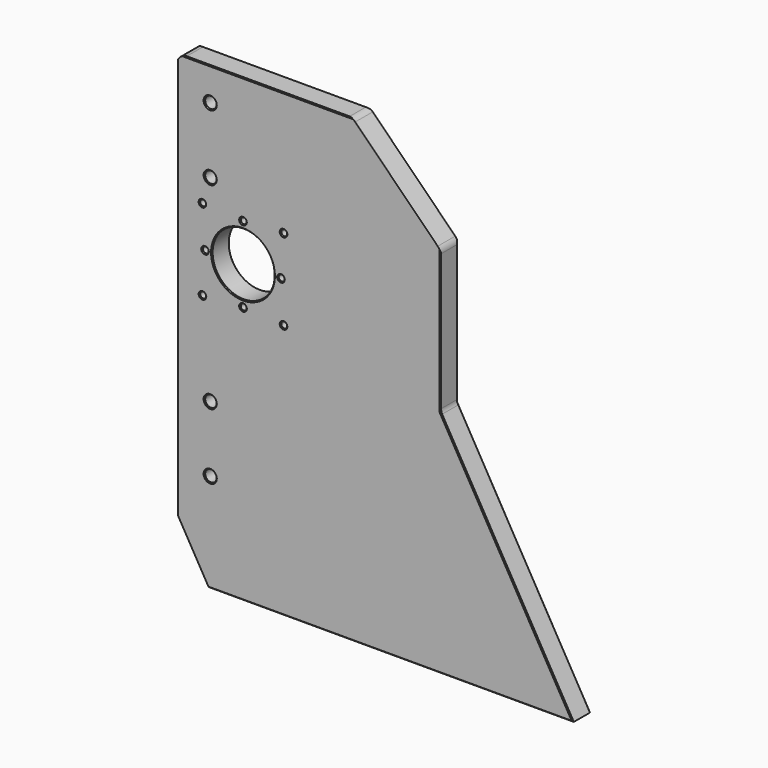
from build123d import *

# Parameters (mm, degrees)
F0_R         = 3.302
F0_R_2       = 1.7
F0_R_3       = 18
F1_DEPTH     = 12.7
F2_SIZE      = 0.508
F3_T1_DEPTH  = 272.9669915773
F4_T4_DEPTH  = 18.4899094878
F4_T10_DEPTH = 18.4899094878
F4_T16_DEPTH = 18.4899094878
F4_T24_DEPTH = 18.4899094878
F4_T30_DEPTH = 18.4899094878
F4_T33_DEPTH = 22.2050244844
F4_T35_DEPTH = 18.4899094878
F4_T37_DEPTH = 37.084


# Not quite as in the source:
# - a fillet or chamfer that OpenCascade refuses, or shapes differently, is made with other operations: its cross-section is extruded or revolved along the edge and cut away or added


with BuildPart() as f1:
    # F0 (on Front) → F1 (new body)
    with BuildSketch(Plane.XZ):
        Polygon((44.9265169831, 0), (44.9265169831, 133.35), (-107.4734830169, 133.35), (-107.4734830169, -102.6728227735), (-89.7620064872, -133.35), (121.9161753795, -133.35), align=None)
        with Locations((-88.4234830169, -76.1876442577)):
            Circle(F0_R, mode=Mode.SUBTRACT)
        with Locations((-88.4234830169, -38.0876442577)):
            Circle(F0_R, mode=Mode.SUBTRACT)
        with Locations((-92.9194827628, 14.6180932346)):
            Circle(F0_R_2, mode=Mode.SUBTRACT)
        with Locations((-69.4244827628, 16.1130932346)):
            Circle(F0_R_2, mode=Mode.SUBTRACT)
        with Locations((-45.9294827628, 14.6180932346)):
            Circle(F0_R_2, mode=Mode.SUBTRACT)
        with Locations((-91.4244827628, 38.1130932346)):
            Circle(F0_R_2, mode=Mode.SUBTRACT)
        with Locations((-69.4244827628, 38.1130932346)):
            Circle(F0_R_3, mode=Mode.SUBTRACT)
        with Locations((-92.9194827628, 61.6080932346)):
            Circle(F0_R_2, mode=Mode.SUBTRACT)
        with Locations((-69.4244827628, 60.1130932346)):
            Circle(F0_R_2, mode=Mode.SUBTRACT)
        with Locations((-47.4244827628, 38.1130932346)):
            Circle(F0_R_2, mode=Mode.SUBTRACT)
        with Locations((-45.9294827628, 61.6080932346)):
            Circle(F0_R_2, mode=Mode.SUBTRACT)
        with Locations((-88.4234830169, 76.2)):
            Circle(F0_R, mode=Mode.SUBTRACT)
        with Locations((-88.4234830169, 114.3)):
            Circle(F0_R, mode=Mode.SUBTRACT)
    extrude(amount=F1_DEPTH)

    # F2
    f2_edges = [f1.edges().sort_by_distance(p)[0] for p in [
        (44.926517, -12.7, 66.675),
        (-31.273483, -12.7, 133.35),
        (-107.473483, -12.7, 15.338589),
        (-98.617745, -12.7, -118.011411),
        (16.077084, -12.7, -133.35),
        (83.421346, -12.7, -66.675),
        (-91.725483, -12.7, -76.187644),
        (-91.725483, -12.7, -38.087644),
        (-94.619483, -12.7, 14.618093),
        (-71.124483, -12.7, 16.113093),
        (-47.629483, -12.7, 14.618093),
        (-93.124483, -12.7, 38.113093),
        (-87.424483, -12.7, 38.113093),
        (-94.619483, -12.7, 61.608093),
        (-71.124483, -12.7, 60.113093),
        (-49.124483, -12.7, 38.113093),
        (-47.629483, -12.7, 61.608093),
        (-91.725483, -12.7, 76.2),
        (-91.725483, -12.7, 114.3),
        (44.926517, 0, 66.675),
        (-31.273483, 0, 133.35),
        (-107.473483, 0, 15.338589),
        (-98.617745, 0, -118.011411),
        (16.077084, 0, -133.35),
        (83.421346, 0, -66.675),
        (-91.725483, 0, -76.187644),
        (-91.725483, 0, -38.087644),
        (-94.619483, 0, 14.618093),
        (-71.124483, 0, 16.113093),
        (-47.629483, 0, 14.618093),
        (-93.124483, 0, 38.113093),
        (-87.424483, 0, 38.113093),
        (-94.619483, 0, 61.608093),
        (-71.124483, 0, 60.113093),
        (-49.124483, 0, 38.113093),
        (-47.629483, 0, 61.608093),
        (-91.725483, 0, 76.2),
        (-91.725483, 0, 114.3),
    ]]
    chamfer(f2_edges, length=F2_SIZE)

    # F3: chamfer of 50.8 on 1 edges, made by hand

    # F3_s2 → F3_t1 (cut)
    with BuildSketch(Plane.XZ.offset(-130.1334957887)):
        Polygon((44.9265169831, 82.55), (-5.8734830169, 133.35), (44.9265169831, 133.35), align=None)
    extrude(amount=F3_T1_DEPTH, mode=Mode.SUBTRACT)

    # F4: fillet of radius 5.08 on 5 edges, made by hand


with BuildPart() as f4_tool2:
    # F4_s3 → F4_t4 (new body)
    with BuildSketch(Plane.XZ.offset(-2.8949547439)):
        with BuildLine():
            ThreePointArc((44.9265169831, 1.3611818976), (45.0996137855, 0.0463811484), (45.6071079319, -1.1788181024))
            Line((45.6071079319, -1.1788181024), (44.9265169831, 0))
            Line((44.9265169831, 0), (44.9265169831, 1.3611818976))
        make_face()
    extrude(amount=F4_T4_DEPTH)

    split(bisect_by=Plane(origin=(22.2092584915, 22.2092584915, 0), x_dir=(0, 0, 1), z_dir=(0.7071067812, 0.7071067812, 0)), keep=Keep.TOP)

    split(bisect_by=Plane(origin=(16.6274734161, 19.1997525055, 9.5998762527), x_dir=(0.755928946, -0.6546536707, 0), z_dir=(-0.6123724357, -0.7071067812, -0.3535533906)), keep=Keep.TOP)


with BuildPart() as f1_1:
    add(f1.part)

    # F4_t1: union F4_tool2
    add(f4_tool2.part)


with BuildPart() as f4_tool8:
    # F4_s9 → F4_t10 (new body)
    with BuildSketch(Plane.XZ.offset(-2.8949547439)):
        with BuildLine():
            ThreePointArc((44.9265169831, 1.3611818976), (45.0996137855, 0.0463811484), (45.6071079319, -1.1788181024))
            Line((45.6071079319, -1.1788181024), (44.9265169831, 0))
            Line((44.9265169831, 0), (44.9265169831, 1.3611818976))
        make_face()
    extrude(amount=F4_T10_DEPTH)

    split(bisect_by=Plane(origin=(22.2092584915, 22.2092584915, 0), x_dir=(0, 0, 1), z_dir=(-0.7071067812, -0.7071067812, 0)), keep=Keep.TOP)

    split(bisect_by=Plane(origin=(16.6274734161, 19.1997525055, 9.5998762527), x_dir=(-0.755928946, 0.6546536707, 0), z_dir=(0.6123724357, 0.7071067812, 0.3535533906)), keep=Keep.TOP)


with BuildPart() as f1_2:
    add(f1_1.part)

    # F4_t7: union F4_tool8
    add(f4_tool8.part)


with BuildPart() as f4_tool14:
    # F4_s15 → F4_t16 (new body)
    with BuildSketch(Plane.XZ.offset(-2.8949547439)):
        with BuildLine():
            ThreePointArc((44.9265169831, 1.3611818976), (45.0996137855, 0.0463811484), (45.6071079319, -1.1788181024))
            Line((45.6071079319, -1.1788181024), (44.9265169831, 0))
            Line((44.9265169831, 0), (44.9265169831, 1.3611818976))
        make_face()
    extrude(amount=F4_T16_DEPTH)

    split(bisect_by=Plane(origin=(22.2092584915, 22.2092584915, 0), x_dir=(0, 0, 1), z_dir=(-0.7071067812, -0.7071067812, 0)), keep=Keep.TOP)

    split(bisect_by=Plane(origin=(28.5592584915, -28.5592584915, 0), x_dir=(0, 0, 1), z_dir=(-0.7071067812, 0.7071067812, 0)), keep=Keep.TOP)

    split(bisect_by=Plane(origin=(16.6274734161, 19.1997525055, 9.5998762527), x_dir=(0.755928946, -0.6546536707, 0), z_dir=(-0.6123724357, -0.7071067812, -0.3535533906)), keep=Keep.TOP)

    split(bisect_by=Plane(origin=(22.1267347301, -25.5497525055, 12.7748762527), x_dir=(-0.755928946, -0.6546536707, 0), z_dir=(-0.6123724357, 0.7071067812, -0.3535533906)), keep=Keep.TOP)


with BuildPart() as f1_3:
    add(f1_2.part)

    # F4_t13: union F4_tool14
    add(f4_tool14.part)


with BuildPart() as f4_tool22:
    # F4_s23 → F4_t24 (new body)
    with BuildSketch(Plane.XZ.offset(-2.8949547439)):
        with BuildLine():
            ThreePointArc((44.9265169831, 1.3611818976), (45.0996137855, 0.0463811484), (45.6071079319, -1.1788181024))
            Line((45.6071079319, -1.1788181024), (44.9265169831, 0))
            Line((44.9265169831, 0), (44.9265169831, 1.3611818976))
        make_face()
    extrude(amount=F4_T24_DEPTH)

    split(bisect_by=Plane(origin=(28.5592584915, -28.5592584915, 0), x_dir=(0, 0, 1), z_dir=(0.7071067812, -0.7071067812, 0)), keep=Keep.TOP)

    split(bisect_by=Plane(origin=(22.1267347301, -25.5497525055, 12.7748762527), x_dir=(-0.755928946, -0.6546536707, 0), z_dir=(-0.6123724357, 0.7071067812, -0.3535533906)), keep=Keep.TOP)


with BuildPart() as f1_4:
    add(f1_3.part)

    # F4_t21: union F4_tool22
    add(f4_tool22.part)


with BuildPart() as f4_tool28:
    # F4_s29 → F4_t30 (new body)
    with BuildSketch(Plane.XZ.offset(-2.8949547439)):
        with BuildLine():
            ThreePointArc((44.9265169831, 1.3611818976), (45.0996137855, 0.0463811484), (45.6071079319, -1.1788181024))
            Line((45.6071079319, -1.1788181024), (44.9265169831, 0))
            Line((44.9265169831, 0), (44.9265169831, 1.3611818976))
        make_face()
    extrude(amount=F4_T30_DEPTH)

    split(bisect_by=Plane(origin=(28.5592584915, -28.5592584915, 0), x_dir=(0, 0, 1), z_dir=(-0.7071067812, 0.7071067812, 0)), keep=Keep.TOP)

    split(bisect_by=Plane(origin=(22.1267347301, -25.5497525055, 12.7748762527), x_dir=(0.755928946, 0.6546536707, 0), z_dir=(0.6123724357, -0.7071067812, 0.3535533906)), keep=Keep.TOP)


with BuildPart() as f1_5:
    add(f1_4.part)

    # F4_t27: union F4_tool28
    add(f4_tool28.part)

    # F4_s34 → F4_t33 (cut)
    with BuildSketch(Plane.XZ.offset(-4.7525122422)):
        with BuildLine():
            ThreePointArc((44.9265169831, 80.4457951032), (44.5398250082, 82.3898269396), (43.4386194315, 84.0378975516))
            Line((43.4386194315, 84.0378975516), (44.9265169831, 82.55))
            Line((44.9265169831, 82.55), (44.9265169831, 80.4457951032))
        make_face()
        with BuildLine():
            ThreePointArc((-4.3855854653, 131.8621024484), (-6.0336560773, 132.9633080252), (-7.9776879138, 133.35))
            Line((-7.9776879138, 133.35), (-5.8734830169, 133.35))
            Line((-5.8734830169, 133.35), (-4.3855854653, 131.8621024484))
        make_face()
    extrude(amount=F4_T33_DEPTH, mode=Mode.SUBTRACT)

    # F4_s36 → F4_t35 (cut)
    with BuildSketch(Plane.XZ.offset(-2.8949547439)):
        with BuildLine():
            ThreePointArc((-107.4734830169, -101.3116408759), (-107.3003862145, -102.626441625), (-106.7928920681, -103.8516408759))
            Line((-106.7928920681, -103.8516408759), (-107.4734830169, -102.6728227735))
            Line((-107.4734830169, -102.6728227735), (-107.4734830169, -101.3116408759))
        make_face()
    extrude(amount=F4_T35_DEPTH, mode=Mode.SUBTRACT)

    # F4_s38 → F4_t37 (cut)
    with BuildSketch(Plane.XZ.offset(-12.192)):
        with BuildLine():
            ThreePointArc((-107.4734830169, 128.27), (-105.9855854653, 131.8621024484), (-102.3934830169, 133.35))
            Line((-102.3934830169, 133.35), (-107.4734830169, 133.35))
            Line((-107.4734830169, 133.35), (-107.4734830169, 128.27))
        make_face()
    extrude(amount=F4_T37_DEPTH, mode=Mode.SUBTRACT)


solid = f1_5.part
